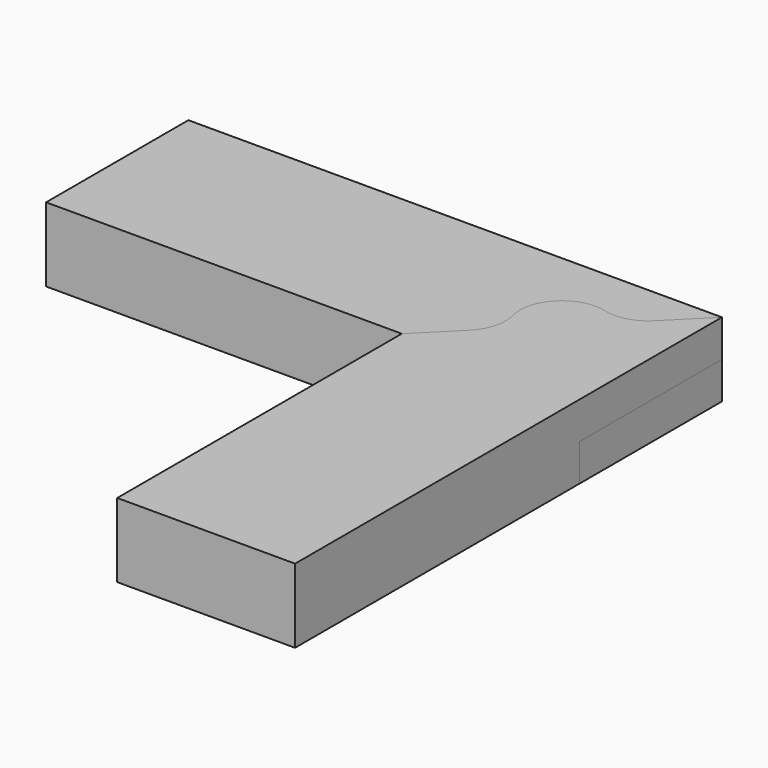
from build123d import *

# Parameters (mm, degrees)
F2_DEPTH = 12.5
F3_W     = 180
F3_H     = 60
F4_DEPTH = 12.5
F6_DEPTH = 12.5
F7_W     = 60
F7_H     = 120
F8_DEPTH = 12.5


with BuildPart() as f2:
    # F1 (on Top) → F2 (new body)
    with BuildSketch(Plane.XY):
        with BuildLine():
            Line((-120, 0), (0, 0))
            Line((0, 0), (12.6794919243, 12.6794919243))
            ThreePointArc((12.6794919243, 12.6794919243), (16.3397459622, 19.0192378865), (16.3397459622, 26.3397459622))
            ThreePointArc((16.3397459622, 26.3397459622), (20, 40), (33.6602540378, 43.6602540378))
            ThreePointArc((33.6602540378, 43.6602540378), (40.9807621135, 43.6602540378), (47.3205080757, 47.3205080757))
            Line((47.3205080757, 47.3205080757), (60, 60))
            Line((60, 60), (-120, 60))
            Line((-120, 60), (-120, 0))
        make_face()
    extrude(amount=F2_DEPTH)

    # F3 (on Top) → F4 (join)
    with BuildSketch(Plane.XY):
        with Locations((-30, 30)):
            Rectangle(F3_W, F3_H)
    extrude(amount=-F4_DEPTH)


with BuildPart() as f6:
    # F5 (on Top) → F6 (new body)
    with BuildSketch(Plane.XY):
        with BuildLine():
            Line((60, -120), (60, 60))
            Line((60, 60), (47.3205080757, 47.3205080757))
            ThreePointArc((47.3205080757, 47.3205080757), (40.9807621135, 43.6602540378), (33.6602540378, 43.6602540378))
            ThreePointArc((33.6602540378, 43.6602540378), (20, 40), (16.3397459622, 26.3397459622))
            ThreePointArc((16.3397459622, 26.3397459622), (16.3397459622, 19.0192378865), (12.6794919243, 12.6794919243))
            Line((12.6794919243, 12.6794919243), (0, 0))
            Line((0, 0), (0, -120))
            Line((0, -120), (60, -120))
        make_face()
    extrude(amount=F6_DEPTH)

    # F7 (on face) → F8 (join)
    with BuildSketch(Plane(origin=(0, 0, 0), x_dir=(1, 0, 0), z_dir=(0, 0, -1))):
        with Locations((30, 60)):
            Rectangle(F7_W, F7_H)
    extrude(amount=F8_DEPTH)


solid = Compound([f2.part, f6.part])
